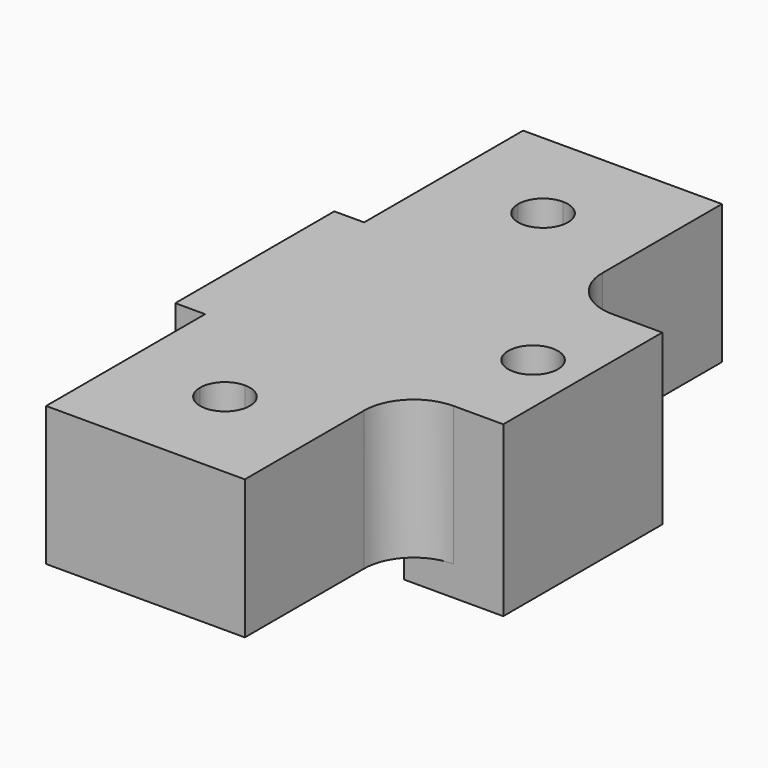
from build123d import *

# Parameters (mm, degrees)
F0_W     = 5
F0_H     = 5
F0_W_2   = 3
F0_H_2   = 20
F0_W_3   = 10
F1_DEPTH = 14
F2_W     = 10
F2_H     = 20
F3_DEPTH = 3
F4_R     = 5
F5_R     = 5
F6_R     = 2.49999
F7_R     = 2.49999
F8_R     = 2.5
F9_DEPTH = 25


# Not quite as in the source:
# - a fillet or chamfer is up to 0.001 mm smaller than in the source, because OpenCascade refuses the exact size


with BuildPart() as f1:
    # F0 (on Top) → F1 (new body)
    with BuildSketch(Plane.XY):
        Polygon((0, 20), (0, 0), (20, 0), (20, 20), (20, 40), (20, 60), (0, 60), (0, 40), align=None)
        with Locations((10, 10)):
            Rectangle(F0_W, F0_H, mode=Mode.SUBTRACT)
        with Locations((10, 50)):
            Rectangle(F0_W, F0_H, mode=Mode.SUBTRACT)
        with Locations((-1.5, 30)):
            Rectangle(F0_W_2, F0_H_2)
        with Locations((25, 30)):
            Rectangle(F0_W_3, F0_H_2)
    extrude(amount=F1_DEPTH)

    # F2 (on face) → F3 (join)
    with BuildSketch(Plane(origin=(0, 0, 0), x_dir=(1, 0, 0), z_dir=(0, 0, -1))):
        with Locations((25, -30)):
            Rectangle(F2_W, F2_H)
    extrude(amount=F3_DEPTH)

    # F4
    f4_edges = [f1.edges().sort_by_distance(p)[0] for p in [
        (20, 40, 7),
    ]]
    fillet(f4_edges, radius=F4_R)

    # F5
    f5_edges = [f1.edges().sort_by_distance(p)[0] for p in [
        (20, 20, 7),
    ]]
    fillet(f5_edges, radius=F5_R)

    # F6 (radius 2.5 in the source; OpenCascade refuses exactly that, so slightly less here)
    f6_edges = [f1.edges().sort_by_distance(p)[0] for p in [
        (7.5, 7.5, 7),
        (7.5, 12.5, 7),
        (12.5, 12.5, 7),
        (12.5, 7.5, 7),
    ]]
    fillet(f6_edges, radius=F6_R)

    # F7 (radius 2.5 in the source; OpenCascade refuses exactly that, so slightly less here)
    f7_edges = [f1.edges().sort_by_distance(p)[0] for p in [
        (12.5, 47.5, 7),
        (7.5, 47.5, 7),
        (7.5, 52.5, 7),
        (12.5, 52.5, 7),
    ]]
    fillet(f7_edges, radius=F7_R)

    # F8 (on face) → F9 (cut)
    with BuildSketch(Plane.XY.offset(14)):
        with Locations((25, 30)):
            Circle(F8_R)
    extrude(amount=-F9_DEPTH, mode=Mode.SUBTRACT)


solid = f1.part
